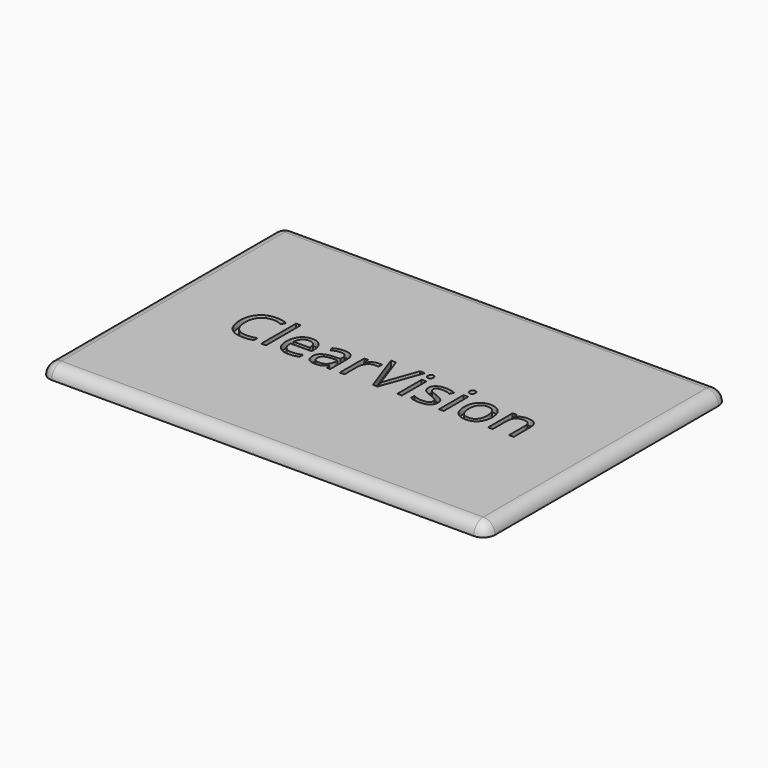
from build123d import *

# Parameters (mm, degrees)
F0_W         = 190.5
F0_H         = 129.54
F1_DEPTH     = 5.08
F2_TEXT_SIZE = 24.471608
F3_DEPTH     = 2.54
F4_R         = 5.07999
F5_T1_DEPTH  = 17.78
F5_T4_ANGLE  = 90
F5_T6_ANGLE  = 90
F5_T8_ANGLE  = 90
F5_T10_ANGLE = 90


# Not quite as in the source:
# - a fillet or chamfer that OpenCascade refuses, or shapes differently, is made with other operations: its cross-section is extruded or revolved along the edge and cut away or added
# - a fillet or chamfer is up to 0.001 mm smaller than in the source, because OpenCascade refuses the exact size
# - Text() gives the source's letters only with a copy of the font that has no kerning and outlines rounded to 1/6400 em; it was checked with that copy


with BuildPart() as f1:
    # F0 (on Top) → F1 (new body)
    with BuildSketch(Plane.XY):
        with Locations((-52.687697, 0.112521)):
            Rectangle(F0_W, F0_H)
    extrude(amount=F1_DEPTH)

    # F2 (on face) → F3 (cut)
    with BuildSketch(Plane.XY.offset(5.08)):
        with Locations((-116.187697, -7.976486)):
            Text('ClearVision', F2_TEXT_SIZE, font='Open Sans', text_align=(TextAlign.LEFT, TextAlign.BOTTOM))
    extrude(amount=-F3_DEPTH, mode=Mode.SUBTRACT)

    # F4 (radius 5.08 in the source; OpenCascade refuses exactly that, so slightly less here)
    f4_edges = [f1.edges().sort_by_distance(p)[0] for p in [
        (-147.937697, 0.112521, 5.08),
        (-52.687697, -64.657479, 5.08),
        (42.562303, 0.112521, 5.08),
        (-52.687697, 64.882521, 5.08),
    ]]
    fillet(f4_edges, radius=F4_R)

    # F5: fillet of radius 5.08 on 4 edges, made by hand

    # F5_s2 → F5_t1 (cut)
    with BuildSketch(Plane.XY.offset(-12.7)):
        with BuildLine():
            ThreePointArc((-142.857697, 64.882521), (-146.449799, 63.394623), (-147.937697, 59.802521))
            Line((-147.937697, 59.802521), (-147.937697, 64.882521))
            Line((-147.937697, 64.882521), (-142.857697, 64.882521))
        make_face()
        with BuildLine():
            ThreePointArc((37.482303, 64.882521), (41.074405, 63.394623), (42.562303, 59.802521))
            Line((42.562303, 59.802521), (42.562303, 64.882521))
            Line((42.562303, 64.882521), (37.482303, 64.882521))
        make_face()
        with BuildLine():
            ThreePointArc((42.562303, -59.577479), (41.074405, -63.169582), (37.482303, -64.657479))
            Line((37.482303, -64.657479), (42.562303, -64.657479))
            Line((42.562303, -64.657479), (42.562303, -59.577479))
        make_face()
        with BuildLine():
            ThreePointArc((-147.937697, -59.577479), (-146.449799, -63.169582), (-142.857697, -64.657479))
            Line((-142.857697, -64.657479), (-147.937697, -64.657479))
            Line((-147.937697, -64.657479), (-147.937697, -59.577479))
        make_face()
    extrude(amount=F5_T1_DEPTH, mode=Mode.SUBTRACT)

    # F5_s3 → F5_t4 (revolve, cut)
    with BuildSketch(Plane.XZ.offset(59.577479)):
        with BuildLine():
            ThreePointArc((-142.857707, 5.08), (-146.449802, 3.592105), (-147.937697, 1e-05))
            Line((-147.937697, 1e-05), (-147.937697, 5.08))
            Line((-147.937697, 5.08), (-142.857707, 5.08))
        make_face()
    revolve(axis=Axis((-142.857697, -59.577479, 5.08), (0, 0, 1)), revolution_arc=F5_T4_ANGLE, mode=Mode.SUBTRACT)

    # F5_s5 → F5_t6 (revolve, cut)
    with BuildSketch(Plane.YZ.offset(37.482303)):
        with BuildLine():
            ThreePointArc((-59.577489, 5.08), (-63.169585, 3.592105), (-64.657479, 1e-05))
            Line((-64.657479, 1e-05), (-64.657479, 5.08))
            Line((-64.657479, 5.08), (-59.577489, 5.08))
        make_face()
    revolve(axis=Axis((37.482303, -59.577479, 5.08), (0, 0, 1)), revolution_arc=F5_T6_ANGLE, mode=Mode.SUBTRACT)

    # F5_s7 → F5_t8 (revolve, cut)
    with BuildSketch(Plane.XZ.offset(-59.802521)):
        with BuildLine():
            ThreePointArc((37.482313, 5.08), (41.074408, 3.592105), (42.562303, 1e-05))
            Line((42.562303, 1e-05), (42.562303, 5.08))
            Line((42.562303, 5.08), (37.482313, 5.08))
        make_face()
    revolve(axis=Axis((37.482303, 59.802521, 5.08), (0, 0, 1)), revolution_arc=F5_T8_ANGLE, mode=Mode.SUBTRACT)

    # F5_s9 → F5_t10 (revolve, cut)
    with BuildSketch(Plane.YZ.offset(-142.857697)):
        with BuildLine():
            ThreePointArc((59.802531, 5.08), (63.394626, 3.592105), (64.882521, 1e-05))
            Line((64.882521, 1e-05), (64.882521, 5.08))
            Line((64.882521, 5.08), (59.802531, 5.08))
        make_face()
    revolve(axis=Axis((-142.857697, 59.802521, 5.08), (0, 0, 1)), revolution_arc=F5_T10_ANGLE, mode=Mode.SUBTRACT)


solid = f1.part
